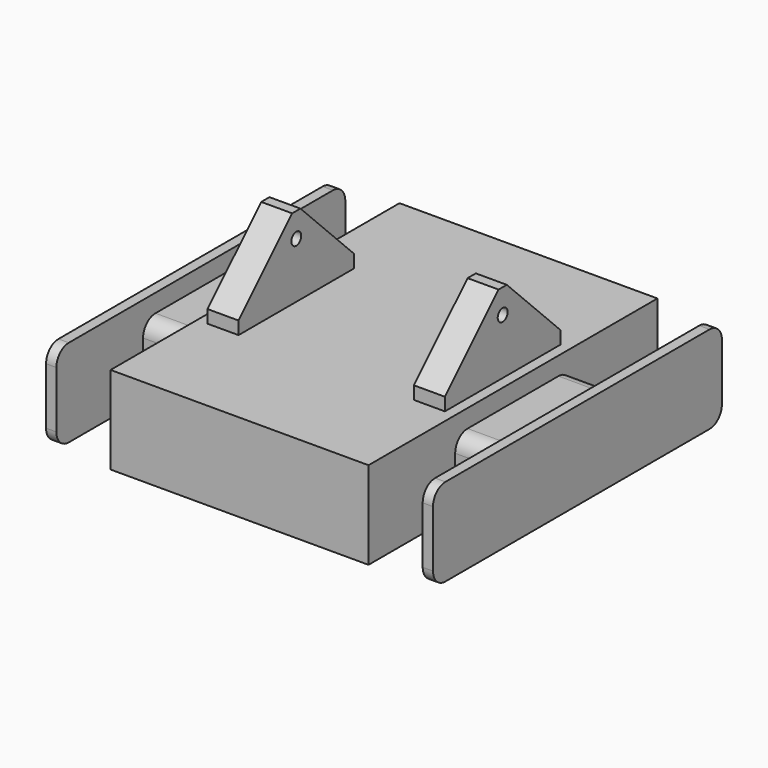
from build123d import *

# Parameters (mm, degrees)
F0_W     = 7.62
F0_H     = 35.56
F1_DEPTH = 10.795
F0_W_2   = 13.335
F2_DEPTH = 6.35
F3_DEPTH = 10.795
F4_DEPTH = 30.48
F5_R     = 3.81
F6_SIZE  = 16.51
F7_R     = 1.524
F8_DEPTH = 76.836
F9_R     = 3.81


# Not quite as in the source:
# - a feature names something its author has since deleted; it is built from what else it names


with BuildPart() as f1:
    # F0 (on Top) → F1 (new body, symmetric)
    with BuildSketch(Plane.XY):
        Polygon((31.75, 44.45), (-31.75, 44.45), (-31.75, 17.78), (-31.75, -17.78), (-31.75, -44.45), (-29.21, -44.45), (31.75, -44.45), (31.75, -31.7187323975), (31.75, -17.78), (31.75, 17.78), align=None)
        with Locations((-25.4, 0)):
            Rectangle(F0_W, F0_H, mode=Mode.SUBTRACT)
        with Locations((25.4, 0)):
            Rectangle(F0_W, F0_H, mode=Mode.SUBTRACT)
    extrude(amount=F1_DEPTH, both=True)



with BuildPart() as f1b:
    # F0 (on Top) → F1, piece 2 (new body, symmetric)
    with BuildSketch(Plane.XY):
        Polygon((-45.085, -17.78), (-45.085, 17.78), (-45.085, 44.45), (-47.625, 44.45), (-47.625, -31.75), (-47.625, -44.45), (-45.085, -44.45), align=None)
    extrude(amount=F1_DEPTH, both=True)


with BuildPart() as f1c:
    # F0 (on Top) → F1, piece 3 (new body, symmetric)
    with BuildSketch(Plane.XY):
        Polygon((45.085, 44.45), (45.085, 17.78), (45.085, -17.78), (45.085, -44.45), (47.625, -44.45), (47.625, -31.75), (47.625, 44.45), align=None)
    extrude(amount=F1_DEPTH, both=True)


with BuildPart() as f1_1:
    add(f1.part)

    add(f1b.part)  # F2 merges F1b

    add(f1c.part)  # F2 merges F1c
    # F0 (on Top) → F2 (join, symmetric)
    with BuildSketch(Plane.XY):
        with Locations((-38.4175, 0)):
            Rectangle(F0_W_2, F0_H)
        with Locations((38.4175, 0)):
            Rectangle(F0_W_2, F0_H)
    extrude(amount=F2_DEPTH, both=True)

    # F0 (on Top) → F3 (join)
    with BuildSketch(Plane.XY):
        with Locations((25.4, 0)):
            Rectangle(F0_W, F0_H)
        with Locations((-25.4, 0)):
            Rectangle(F0_W, F0_H)
    extrude(amount=-F3_DEPTH)

    # F0 (on Top) → F4 (join)
    with BuildSketch(Plane.XY):
        with Locations((25.4, 0)):
            Rectangle(F0_W, F0_H)
        with Locations((-25.4, 0)):
            Rectangle(F0_W, F0_H)
    extrude(amount=F4_DEPTH)

    # F5
    f5_edges = [f1_1.edges().sort_by_distance(p)[0] for p in [
        (38.4175, -17.78, 6.35),
        (38.4175, -17.78, -6.35),
        (38.4175, 17.78, 6.35),
        (38.4175, 17.78, -6.35),
        (-38.4175, 17.78, -6.35),
        (-38.4175, -17.78, -6.35),
        (-38.4175, 17.78, 6.35),
        (-38.4175, -17.78, 6.35),
    ]]
    fillet(f5_edges, radius=F5_R)

    # F6
    f6_edges = [f1_1.edges().sort_by_distance(p)[0] for p in [
        (25.4, 17.78, 30.48),
        (-25.4, 17.78, 30.48),
        (25.4, -17.78, 30.48),
        (-25.4, -17.78, 30.48),
    ]]
    chamfer(f6_edges, length=F6_SIZE)

    # F7 (on face) → F8 (cut, through all)
    with BuildSketch(Plane.YZ.offset(29.21)):
        with Locations((0, 24.4627408683)):
            Circle(F7_R)
    extrude(amount=-F8_DEPTH, mode=Mode.SUBTRACT)

    # F9
    f9_edges = [f1_1.edges().sort_by_distance(p)[0] for p in [
        (46.355, 44.45, 10.795),
        (-46.355, 44.45, 10.795),
        (-46.355, 44.45, -10.795),
        (46.355, 44.45, -10.795),
        (-46.355, -44.45, 10.795),
        (-46.355, -44.45, -10.795),
        (46.355, -44.45, -10.795),
        (46.355, -44.45, 10.795),
    ]]
    fillet(f9_edges, radius=F9_R)


solid = f1_1.part
